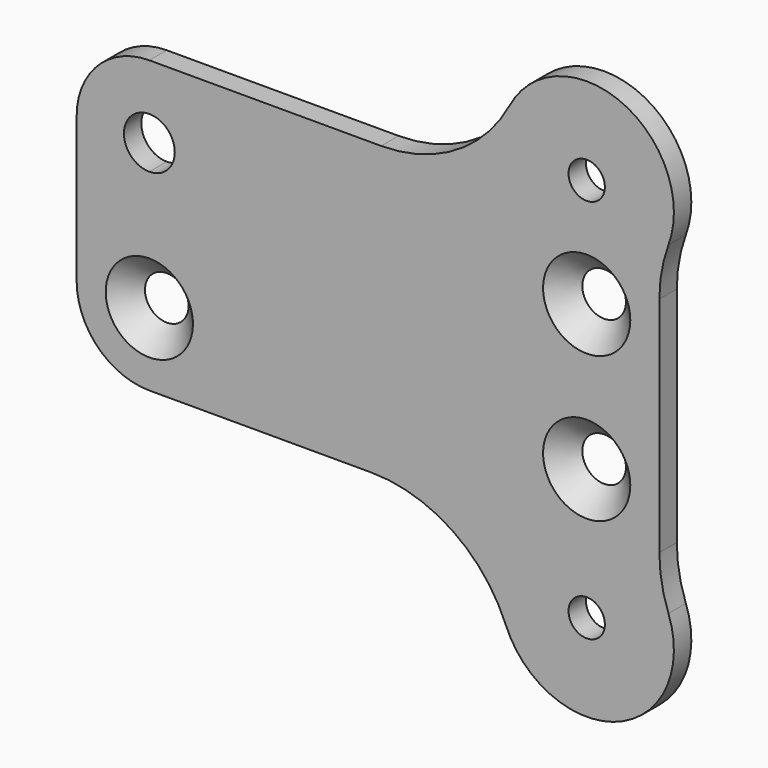
from build123d import *

# Parameters (mm, degrees)
F0_R     = 2.5
F1_DEPTH = 3


# Not quite as in the source:
# - a fillet or chamfer that OpenCascade refuses, or shapes differently, is made with other operations: its cross-section is extruded or revolved along the edge and cut away or added


with BuildPart() as f1:
    # F0 (on Front) → F1 (new body)
    with BuildSketch(Plane.XZ):
        with BuildLine():
            Line((40.1844298095, -16.8644712743), (40.1844298095, 13.8644712743))
            ThreePointArc((40.1844298095, 13.8644712743), (40.4994101244, 17.4000051803), (41.4344298095, 20.8241767279))
            ThreePointArc((41.4344298095, 20.8241767279), (35.0877662109, 35.9525016382), (19.5764143341, 30.6098135152))
            ThreePointArc((19.5764143341, 30.6098135152), (12.2164228481, 22.827751719), (1.8963885419, 19.9595027072))
            Line((1.8963885419, 19.9595027072), (-30, 19.9595027072))
            ThreePointArc((-30, 19.9595027072), (-37.0710678119, 17.030570519), (-40, 9.9595027072))
            Line((-40, 9.9595027072), (-40, -10.0404972928))
            ThreePointArc((-40, -10.0404972928), (-37.0710678119, -17.1115651047), (-30, -20.0404972928))
            Line((-30, -20.0404972928), (0.5360500065, -20.0404972928))
            ThreePointArc((0.5360500065, -20.0404972928), (11.7050648207, -23.4497436005), (19.0662873833, -32.5151864848))
            ThreePointArc((19.0662873833, -32.5151864848), (34.5304347857, -39.18535832), (41.4344298095, -23.8241767279))
            ThreePointArc((41.4344298095, -23.8241767279), (40.4994101244, -20.4000051803), (40.1844298095, -16.8644712743))
        make_face()
        with BuildLine():
            ThreePointArc((-30, -7.5404972928), (-28.232233047, -8.2727303399), (-27.5, -10.0404972928))
            ThreePointArc((-27.5, -10.0404972928), (-31.767766953, -11.8082642458), (-30, -7.5404972928))
        make_face(mode=Mode.SUBTRACT)
        with Locations((30.1844298095, -28)):
            Circle(F0_R, mode=Mode.SUBTRACT)
        with Locations((30.1844298095, -10)):
            Circle(F0_R, mode=Mode.SUBTRACT)
        with BuildLine():
            ThreePointArc((-26.5, 9.9595027072), (-27.5251262658, 7.484628973), (-30, 6.4595027072))
            ThreePointArc((-30, 6.4595027072), (-32.4748737342, 12.4343764413), (-26.5, 9.9595027072))
        make_face(mode=Mode.SUBTRACT)
        with Locations((30.1844298095, 10)):
            Circle(F0_R, mode=Mode.SUBTRACT)
        with Locations((30.1844298095, 25)):
            Circle(F0_R, mode=Mode.SUBTRACT)
    extrude(amount=F1_DEPTH)

    # F2: chamfer of 3.5 on 3 edges, made by hand

    # F2_s1 → F2_t2 (revolve, cut)
    with BuildSketch(Plane.YZ.offset(-30)):
        Polygon((-3, -4.0404972928), (0.5, -7.5404972928), (-3, -7.5404972928), align=None)
    revolve(axis=Axis((-30, -3, -10.0404972928), (0, -1, 0)), mode=Mode.SUBTRACT)

    # F2_s3 → F2_t4 (revolve, cut)
    with BuildSketch(Plane.XY.offset(-10)):
        Polygon((36.1844298095, -3), (32.6844298095, 0.5), (32.6844298095, -3), align=None)
    revolve(axis=Axis((30.1844298095, -3, -10), (0, -1, 0)), mode=Mode.SUBTRACT)

    # F2_s5 → F2_t6 (revolve, cut)
    with BuildSketch(Plane.XY.offset(10)):
        Polygon((36.1844298095, -3), (32.6844298095, 0.5), (32.6844298095, -3), align=None)
    revolve(axis=Axis((30.1844298095, -3, 10), (0, -1, 0)), mode=Mode.SUBTRACT)


solid = f1.part
